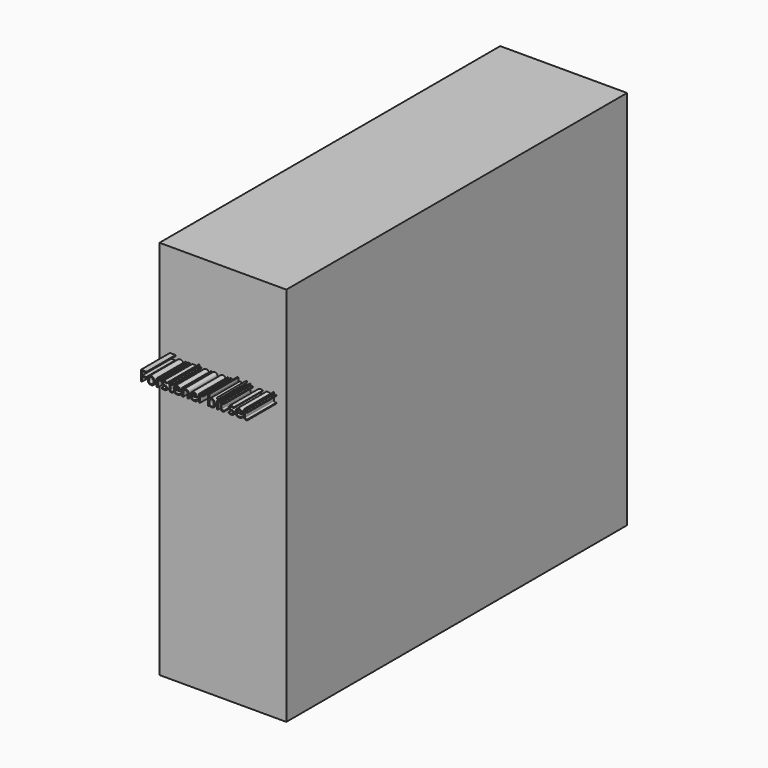
from build123d import *

# Parameters (mm, degrees)
F0_W         = 88.9
F0_H         = 266.7
F1_DEPTH     = 298.45
F2_TEXT_SIZE = 9.9269240947
F3_DEPTH     = 25.4


# Not quite as in the source:
# - Text() gives the source's letters only with a copy of the font that has no kerning and outlines rounded to 1/6400 em; it was checked with that copy


with BuildPart() as f1:
    # F0 (on Front) → F1 (new body)
    with BuildSketch(Plane.XZ):
        Rectangle(F0_W, F0_H)
    extrude(amount=F1_DEPTH)

    # F2 (on face) → F3 (join)
    with BuildSketch(Plane.XZ.offset(298.45)):
        with Locations((-38.1, 60.6690839204)):
            Text('Forstener bit set', F2_TEXT_SIZE, font='Open Sans', text_align=(TextAlign.LEFT, TextAlign.BOTTOM))
    extrude(amount=F3_DEPTH)


solid = f1.part
